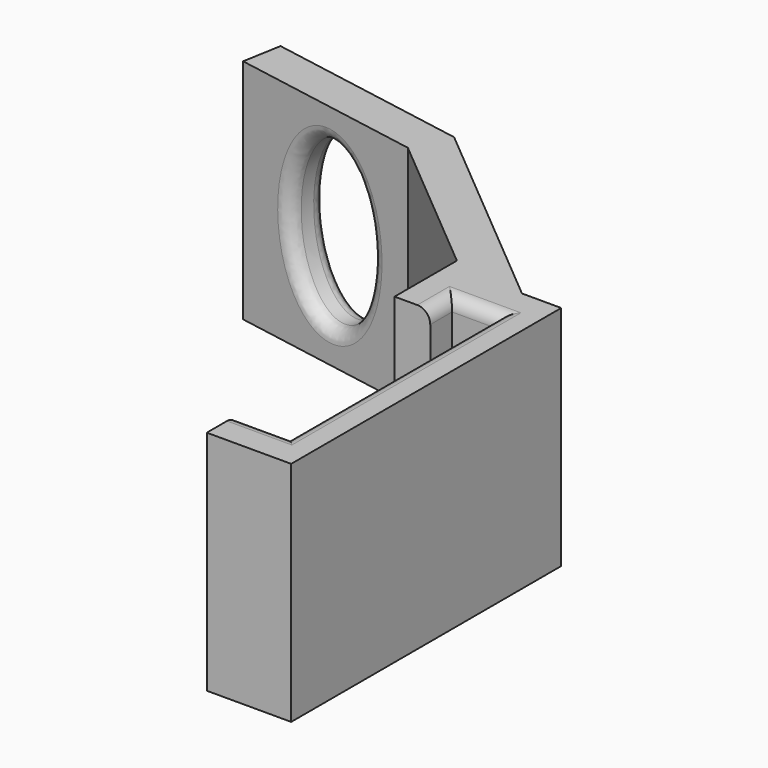
from build123d import *

# Parameters (mm, degrees)
F1_DEPTH = 35
F3_DEPTH = 25
F4_R     = 2
F5_R     = 2


with BuildPart() as f1:
    # F0 (on Top) → F1 (new body)
    with BuildSketch(Plane.XY):
        Polygon((8, 5.8818385005), (0, 5.8818385005), (0, 0), (13, 0), (13, 52), (6.9578553956, 52), (-24.8561735749, 78.6951399753), (-55.9836768179, 84.1837586392), (-57.0255658839, 78.2749121211), (-27.4813332936, 73.0654667911), (-4.5, 53.7818385005), (-4.5, 41.7818385005), (1, 41.7818385005), (1, 45.9818385005), (8, 45.9818385005), align=None)
    extrude(amount=F1_DEPTH)

    # F2 (on face) → F3 (cut)
    with BuildSketch(Plane(origin=(12.7081561839, 72.0715351266, 0), x_dir=(-0.984807753, 0.1736481777, 0), z_dir=(0.1736481777, 0.984807753, 0))):
        with BuildLine():
            add(Edge.make_bspline(
                [(53.947667672, 30), (40.9572866152, 30), (47.4524771436, 11.25), (53.947667672, -7.5), (60.4428582004, 11.25), (66.9380487288, 30), (53.947667672, 30)],
                knots=[0, 0, 0, 2.0943951024, 2.0943951024, 4.1887902048, 4.1887902048, 6.2831853072, 6.2831853072, 6.2831853072], degree=2, weights=[1, 0.5, 1, 0.5, 1, 0.5, 1]))
        make_face()
    extrude(amount=-F3_DEPTH, mode=Mode.SUBTRACT)

    # F4
    f4_edges = [f1.edges().sort_by_distance(p)[0] for p in [
        (4.5, 45.981839, 35),
        (8, 25.931839, 35),
        (4, 5.881839, 35),
        (1, 43.881839, 35),
        (4, 5.881839, 0),
        (8, 25.931839, 0),
        (4.5, 45.981839, 0),
        (1, 43.881839, 0),
    ]]
    fillet(f4_edges, radius=F4_R)

    # F5
    f5_edges = [f1.edges().sort_by_distance(p)[0] for p in [
        (-40.419925, 81.439449, 5),
        (-41.461814, 75.530603, 5),
    ]]
    fillet(f5_edges, radius=F5_R)


solid = f1.part
